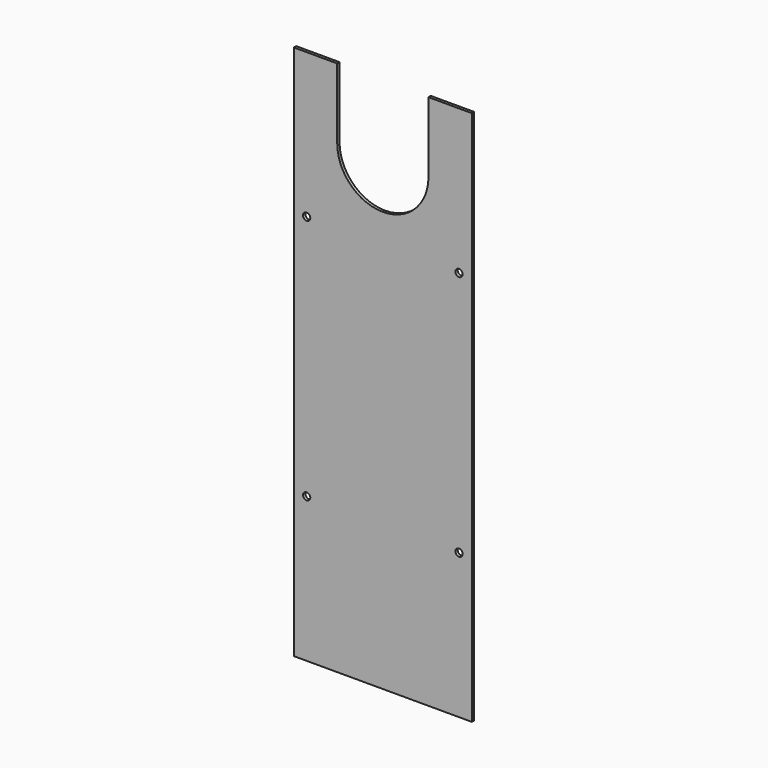
from build123d import *

# Parameters (mm, degrees)
F0_R     = 2.5
F1_DEPTH = 2
F2_R     = 31.49999


# Not quite as in the source:
# - a fillet or chamfer is up to 0.001 mm smaller than in the source, because OpenCascade refuses the exact size


with BuildPart() as f1:
    # F0 (on Front) → F1 (new body)
    with BuildSketch(Plane.XZ):
        Polygon((-61.5, 0), (0, 0), (61.5, 0), (61.5, 370), (31.5, 370), (31.5, 290), (5.5, 290), (-5.5, 290), (-31.5, 290), (-31.5, 370), (-61.5, 370), align=None)
        with Locations((-52.6, 100)):
            Circle(F0_R, mode=Mode.SUBTRACT)
        with Locations((52.6, 100)):
            Circle(F0_R, mode=Mode.SUBTRACT)
        with Locations((-52.6, 270)):
            Circle(F0_R, mode=Mode.SUBTRACT)
        with Locations((52.6, 270)):
            Circle(F0_R, mode=Mode.SUBTRACT)
    extrude(amount=F1_DEPTH)

    # F2 (radius 31.5 in the source; OpenCascade refuses exactly that, so slightly less here)
    f2_edges = [f1.edges().sort_by_distance(p)[0] for p in [
        (-31.5, -1, 290),
        (31.5, -1, 290),
    ]]
    fillet(f2_edges, radius=F2_R)


solid = f1.part
